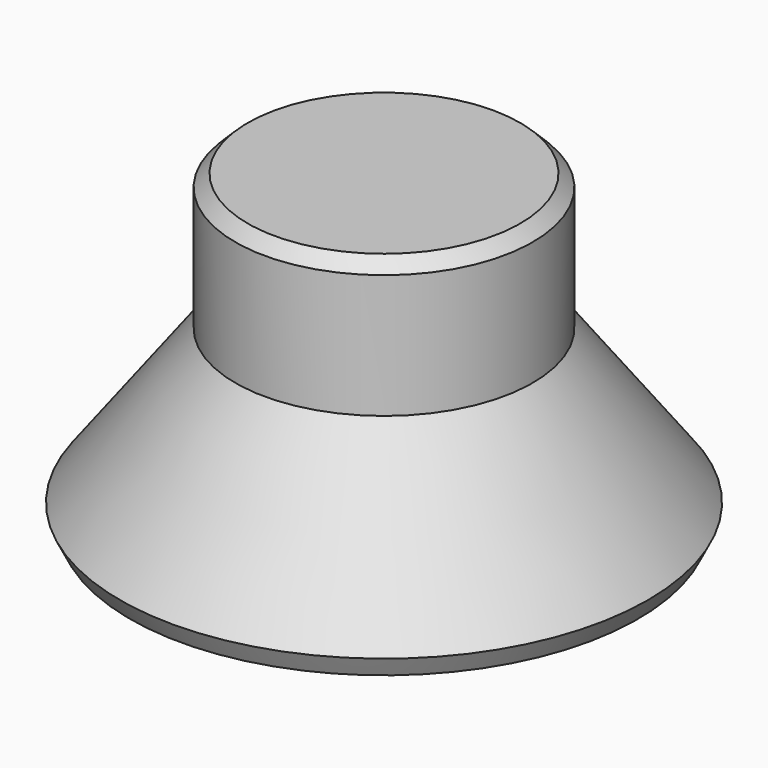
from build123d import *


# Not quite as in the source:
# - a fillet or chamfer that OpenCascade refuses, or shapes differently, is made with other operations: its cross-section is extruded or revolved along the edge and cut away or added


with BuildPart() as f1:
    # F0 (on Right) → F1 (revolve)
    with BuildSketch(Plane.YZ):
        Polygon((0, 50), (0, 0), (45, 0), (24, 28), (24, 50), align=None)
    revolve(axis=Axis((0, 0, 9.18032974), (0, 0, -1)))

    # F2: chamfer of 2 on 2 edges, made by hand

    # F2_s1 → F2_t2 (revolve, cut)
    with BuildSketch(Plane.YZ):
        Polygon((24, 48), (22, 50), (24, 50), align=None)
    revolve(axis=Axis((0, 0, 50), (0, 0, -1)), mode=Mode.SUBTRACT)

    # F2_s3 → F2_t4 (revolve, cut)
    with BuildSketch(Plane.YZ):
        Polygon((41, 0), (42.6, 3.2), (45, 0), align=None)
    revolve(axis=Axis((0, 0, 0), (0, 0, -1)), mode=Mode.SUBTRACT)


solid = f1.part
